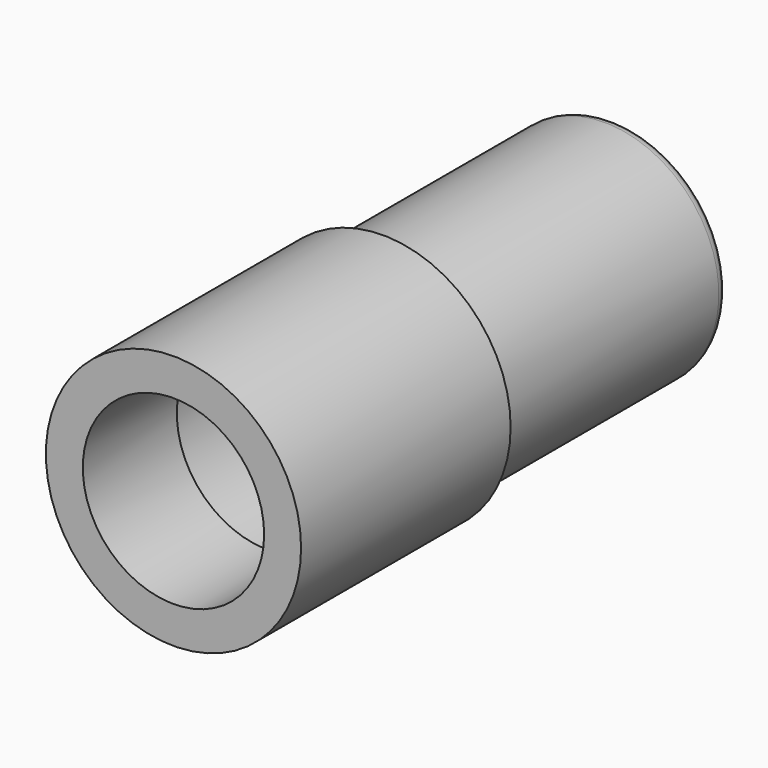
from build123d import *

# Parameters (mm, degrees)
F0_R     = 9.652
F0_R_2   = 6.858
F1_DEPTH = 3.302
F2_R     = 9.652
F2_R_2   = 8.001
F3_DEPTH = 7.62
F4_R     = 9.652
F4_R_2   = 8.001
F4_R_3   = 6.858
F5_DEPTH = 8.89
F6_R     = 8.636
F6_R_2   = 6.858
F7_DEPTH = 21.844
F8_R     = 0.88899


# Not quite as in the source:
# - a fillet or chamfer is up to 0.001 mm smaller than in the source, because OpenCascade refuses the exact size


with BuildPart() as f1:
    # F0 (on Front) → F1 (new body)
    with BuildSketch(Plane.XZ):
        Circle(F0_R)
        Circle(F0_R_2, mode=Mode.SUBTRACT)
    extrude(amount=F1_DEPTH)

    # F2 (on face) → F3 (join)
    with BuildSketch(Plane.XZ.offset(3.302)):
        Circle(F2_R)
        Circle(F2_R_2, mode=Mode.SUBTRACT)
    extrude(amount=F3_DEPTH)

    # F4 (on face) → F5 (join)
    with BuildSketch(Plane.XZ.offset(10.922)):
        Circle(F4_R)
        Circle(F4_R_2, mode=Mode.SUBTRACT)
        Circle(F4_R_2)
        Circle(F4_R_3, mode=Mode.SUBTRACT)
    extrude(amount=F5_DEPTH)

    # F6 (on face) → F7 (join)
    with BuildSketch(Plane(origin=(0, 0, 0), x_dir=(-1, 0, 0), z_dir=(0, 1, 0))):
        Circle(F6_R)
        Circle(F6_R_2, mode=Mode.SUBTRACT)
    extrude(amount=F7_DEPTH)

    # F8 (radius 0.889 in the source; OpenCascade refuses exactly that, so slightly less here)
    f8_edges = [f1.edges().sort_by_distance(p)[0] for p in [
        (6.858, 21.844, 0),
        (8.636, 21.844, 0),
    ]]
    fillet(f8_edges, radius=F8_R)


solid = f1.part
